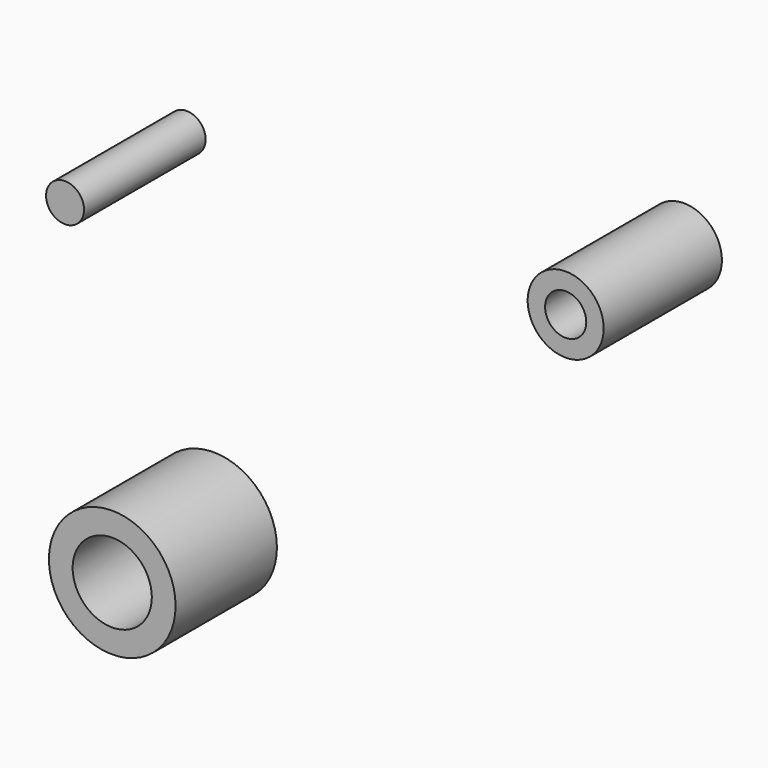
from build123d import *

# Parameters (mm, degrees)
F0_R      = 2.38125
F1_DEPTH  = 19.05
F2_R      = 4.7625
F2_R_2    = 2.5796875
F3_DEPTH  = 15.35
F2_R_3    = 1.5875
F4_DEPTH  = 3.175
F5_SIZE   = 0.79375
F6_R      = 7.9375
F6_R_2    = 4.9609375
F7_DEPTH  = 12.7
F6_R_3    = 4.7625
F6_R_4    = 2.778125
F8_DEPTH  = 3.175
F9_DEPTH  = 3.175
F10_D     = 1.9939
F10_DEPTH = 3.175
F10_TIP   = 0.5990279941


# Not quite as in the source:
# - a length typed as a fraction of an inch, garbled in the dataset ("3 / 203.2 mm" for 3/8 in), is restored


with BuildPart() as f1:
    # F0 (on Front) → F1 (new body)
    with BuildSketch(Plane.XZ):
        with Locations((-39.3053889275, 31.8004786968)):
            Circle(F0_R)
    extrude(amount=F1_DEPTH)

    # F10
    with Locations(Plane(origin=(0, 0, 0), x_dir=(1, 0, 0), z_dir=(0, 1, 0))):
        with Locations((-39.3053889275, -31.8004786968)):
            Hole(F10_D / 2, depth=F10_DEPTH)
            with Locations((0, 0, -(F10_DEPTH + F10_TIP / 2))):  # 118° drill point
                Cone(0, F10_D / 2, F10_TIP, mode=Mode.SUBTRACT)


with BuildPart() as f3:
    # F2 (on Front) → F3 (new body)
    with BuildSketch(Plane.XZ):
        with Locations((20.4795077443, 37.3973622918)):
            Circle(F2_R)
        with Locations((20.4795077443, 37.3973622918)):
            Circle(F2_R_2, mode=Mode.SUBTRACT)
    extrude(amount=F3_DEPTH)

    # F2 (on Front) → F4 (join)
    with BuildSketch(Plane.XZ):
        with Locations((20.4795077443, 37.3973622918)):
            Circle(F2_R)
        with Locations((20.4795077443, 37.3973622918)):
            Circle(F2_R_2, mode=Mode.SUBTRACT)
        with Locations((20.4795077443, 37.3973622918)):
            Circle(F2_R_2)
        with Locations((20.4795077443, 37.3973622918)):
            Circle(F2_R_3, mode=Mode.SUBTRACT)
    extrude(amount=-F4_DEPTH)

    # F5
    f5_edges = [f3.edges().sort_by_distance(p)[0] for p in [
        (18.892008, 3.175, 37.397362),
    ]]
    chamfer(f5_edges, length=F5_SIZE)


with BuildPart() as f7:
    # F6 (on Front) → F7 (new body)
    with BuildSketch(Plane.XZ):
        with Locations((-38.4694747627, -12.4227562919)):
            Circle(F6_R)
        with Locations((-38.4694747627, -12.4227562919)):
            Circle(F6_R_2, mode=Mode.SUBTRACT)
    extrude(amount=F7_DEPTH)

    # F6 (on Front) → F8 (join)
    with BuildSketch(Plane.XZ):
        with Locations((-38.4694747627, -12.4227562919)):
            Circle(F6_R)
        with Locations((-38.4694747627, -12.4227562919)):
            Circle(F6_R_2, mode=Mode.SUBTRACT)
        with Locations((-38.4694747627, -12.4227562919)):
            Circle(F6_R_2)
        with Locations((-38.4694747627, -12.4227562919)):
            Circle(F6_R_3, mode=Mode.SUBTRACT)
        with Locations((-38.4694747627, -12.4227562919)):
            Circle(F6_R_3)
        with Locations((-38.4694747627, -12.4227562919)):
            Circle(F6_R_4, mode=Mode.SUBTRACT)
    extrude(amount=-F8_DEPTH)

    # F6 (on Front) → F9 (join)
    with BuildSketch(Plane.XZ):
        with Locations((-38.4694747627, -12.4227562919)):
            Circle(F6_R_2)
        with Locations((-38.4694747627, -12.4227562919)):
            Circle(F6_R_3, mode=Mode.SUBTRACT)
    extrude(amount=F9_DEPTH)


solid = Compound([f1.part, f3.part, f7.part])
